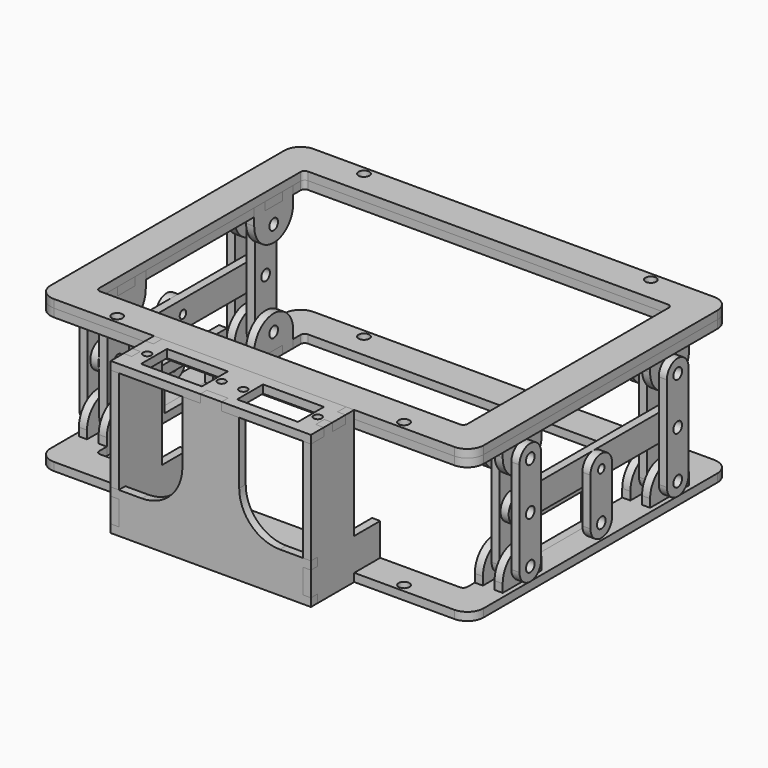
from build123d import *

# Parameters (mm, degrees)
F0_W           = 160
F0_H           = 120
F0_W_2         = 136
F0_H_2         = 96
F1_DEPTH       = 3
F2_R           = 6
F3_R           = 1.5
F4_R           = 2
F5_DEPTH       = 3.001
F6_W           = 2.9
F6_H           = 4.9
F7_DEPTH       = 3.001
F8_R           = 2
F9_DEPTH       = 3
F10_R          = 2
F11_DEPTH      = 3
F18_R          = 2
F19_DEPTH      = 3
F24_R          = 2
F25_DEPTH      = 7
F26_DEPTH      = 4
F30_R          = 1.5
F31_DEPTH      = 158.601
F32_W          = 35.5
F32_H          = 19
F32_R          = 1.5
F32_W_2        = 22.5
F32_H_2        = 12
F33_DEPTH      = 3
F34_W          = 35.3
F34_H          = 3
F35_DEPTH      = 2.9
F35_DEPTH_BACK = 138.9
F36_R          = 2
F36_R_2        = 1.5
F37_DEPTH      = 3
F38_R          = 1.5
F38_W          = 22.5
F38_H          = 12
F39_DEPTH      = 3
F41_DEPTH      = 3
F42_R          = 15
F44_DEPTH      = 3
F45_W          = 3
F45_H          = 4
F46_DEPTH      = 3
F48_R          = 3


with BuildPart() as f1:
    # F0 (on Top) → F1 (new body)
    with BuildSketch(Plane.XY):
        with Locations((-83.0341556995, -58.1203717301)):
            Rectangle(F0_W, F0_H)
        with Locations((-83.0341556995, -58.1203717301)):
            Rectangle(F0_W_2, F0_H_2, mode=Mode.SUBTRACT)
    extrude(amount=F1_DEPTH)

    # F2
    f2_edges = [f1.edges().sort_by_distance(p)[0] for p in [
        (-163.034156, -118.120372, 1.5),
        (-3.034156, -118.120372, 1.5),
        (-163.034156, 1.879628, 1.5),
        (-3.034156, 1.879628, 1.5),
    ]]
    fillet(f2_edges, radius=F2_R)

    # F3
    f3_edges = [f1.edges().sort_by_distance(p)[0] for p in [
        (-151.034156, -10.120372, 1.5),
        (-15.034156, -10.120372, 1.5),
        (-15.034156, -106.120372, 1.5),
        (-151.034156, -106.120372, 1.5),
    ]]
    fillet(f3_edges, radius=F3_R)

    # F4 (on face) → F5 (cut, through all)
    with BuildSketch(Plane.XY.offset(3)):
        with Locations((-136.0341556995, -1.1203717301)):
            Circle(F4_R)
        with Locations((-30.0341556995, -1.1203717301)):
            Circle(F4_R)
        with Locations((-30.0341556995, -115.1203717301)):
            Circle(F4_R)
        with Locations((-136.0341556995, -115.1203717301)):
            Circle(F4_R)
    extrude(amount=-F5_DEPTH, mode=Mode.SUBTRACT)

    # F6 (on face) → F7 (cut, through all)
    with BuildSketch(Plane.XY.offset(3)):
        with Locations((-152.4841556995, -98.6703717301)):
            Rectangle(F6_W, F6_H)
        with Locations((-152.4841556995, -85.6703717301)):
            Rectangle(F6_W, F6_H)
        with Locations((-159.8841556995, -98.6703717301)):
            Rectangle(F6_W, F6_H)
        with Locations((-159.8841556995, -85.6703717301)):
            Rectangle(F6_W, F6_H)
        with Locations((-6.1841556995, -98.6703717301)):
            Rectangle(F6_W, F6_H)
        with Locations((-6.1841556995, -85.6703717301)):
            Rectangle(F6_W, F6_H)
        with Locations((-13.5841556995, -85.6703717301)):
            Rectangle(F6_W, F6_H)
        with Locations((-13.5841556995, -98.6703717301)):
            Rectangle(F6_W, F6_H)
        with Locations((-6.1841556995, -17.5703717301)):
            Rectangle(F6_W, F6_H)
        with Locations((-152.4841556995, -17.5703717301)):
            Rectangle(F6_W, F6_H)
        with Locations((-13.5841556995, -17.5703717301)):
            Rectangle(F6_W, F6_H)
        with Locations((-159.8841556995, -30.5703717301)):
            Rectangle(F6_W, F6_H)
        with Locations((-159.8841556995, -17.5703717301)):
            Rectangle(F6_W, F6_H)
        with Locations((-13.5841556995, -30.5703717301)):
            Rectangle(F6_W, F6_H)
        with Locations((-6.1841556995, -30.5703717301)):
            Rectangle(F6_W, F6_H)
        with Locations((-152.4841556995, -30.5703717301)):
            Rectangle(F6_W, F6_H)
    extrude(amount=-F7_DEPTH, mode=Mode.SUBTRACT)


with BuildPart() as f9:
    # F8 (on face) → F9 (new body)
    with BuildSketch(Plane.XY.offset(3)):
        with BuildLine():
            ThreePointArc((-3.0341556995, -4.1203717301), (-4.7915150124, 0.122268957), (-9.0341556995, 1.8796282699))
            Line((-9.0341556995, 1.8796282699), (-157.0341556995, 1.8796282699))
            ThreePointArc((-157.0341556995, 1.8796282699), (-161.2767963867, 0.122268957), (-163.0341556995, -4.1203717301))
            Line((-163.0341556995, -4.1203717301), (-163.0341556995, -112.1203717301))
            ThreePointArc((-163.0341556995, -112.1203717301), (-161.2767963867, -116.3630124172), (-157.0341556995, -118.1203717301))
            Line((-157.0341556995, -118.1203717301), (-9.0341556995, -118.1203717301))
            ThreePointArc((-9.0341556995, -118.1203717301), (-4.7915150124, -116.3630124172), (-3.0341556995, -112.1203717301))
            Line((-3.0341556995, -112.1203717301), (-3.0341556995, -4.1203717301))
        make_face()
        with Locations((-136.0341556995, -115.1203717301)):
            Circle(F8_R, mode=Mode.SUBTRACT)
        with Locations((-30.0341556995, -115.1203717301)):
            Circle(F8_R, mode=Mode.SUBTRACT)
        with Locations((-136.0341556995, -1.1203717301)):
            Circle(F8_R, mode=Mode.SUBTRACT)
        with BuildLine():
            Line((-16.5341556995, -106.1203717301), (-149.5341556995, -106.1203717301))
            ThreePointArc((-149.5341556995, -106.1203717301), (-150.5948158713, -105.6810319019), (-151.0341556995, -104.6203717301))
            Line((-151.0341556995, -104.6203717301), (-151.0341556995, -11.6203717301))
            ThreePointArc((-151.0341556995, -11.6203717301), (-150.5948158713, -10.5597115583), (-149.5341556995, -10.1203717301))
            Line((-149.5341556995, -10.1203717301), (-16.5341556995, -10.1203717301))
            ThreePointArc((-16.5341556995, -10.1203717301), (-15.4734955278, -10.5597115583), (-15.0341556995, -11.6203717301))
            Line((-15.0341556995, -11.6203717301), (-15.0341556995, -104.6203717301))
            ThreePointArc((-15.0341556995, -104.6203717301), (-15.4734955278, -105.6810319019), (-16.5341556995, -106.1203717301))
        make_face(mode=Mode.SUBTRACT)
        with Locations((-30.0341556995, -1.1203717301)):
            Circle(F8_R, mode=Mode.SUBTRACT)
    extrude(amount=F9_DEPTH)


with BuildPart() as f11:
    # F10 (on face) → F11 (new body)
    with BuildSketch(Plane.YZ.offset(-151.0341556995)):
        with BuildLine():
            Line((-96.2203717301, 3), (-101.1703717301, 3))
            Line((-101.1703717301, 3), (-101.1703717301, -3))
            ThreePointArc((-101.1703717301, -3), (-92.1703717301, -12), (-83.1703717301, -3))
            Line((-83.1703717301, -3), (-83.1703717301, 3))
            Line((-83.1703717301, 3), (-88.1203717301, 3))
            Line((-88.1203717301, 3), (-88.1203717301, 0))
            Line((-88.1203717301, 0), (-88.1703717301, 0))
            Line((-88.1703717301, 0), (-96.1703717301, 0))
            Line((-96.1703717301, 0), (-96.2203717301, 0))
            Line((-96.2203717301, 0), (-96.2203717301, 3))
        make_face()
        with Locations((-92.1703717301, -6)):
            Circle(F10_R, mode=Mode.SUBTRACT)
    extrude(amount=-F11_DEPTH)


with BuildPart() as f13_1:
    # F13: instance of F11
    add(f11.part.mirror(Plane(origin=(-156.1841556995, -71.8953717301, 1.5), x_dir=(0, 1, 0), z_dir=(1, 0, 0))))


with BuildPart() as f16_1:
    # F16: instance of F11
    add(f11.part.mirror(Plane(origin=(-83.0341556995, -58.1203717301, 1.5), x_dir=(0, 1, 0), z_dir=(1, 0, 0))))


with BuildPart() as f16_2:
    # F16: instance of F13_1
    add(f13_1.part.mirror(Plane(origin=(-83.0341556995, -58.1203717301, 1.5), x_dir=(0, 1, 0), z_dir=(1, 0, 0))))


with BuildPart() as f17_1:
    # F17: instance of F11
    add(f11.part.mirror(Plane(origin=(-83.0341556995, -58.1203717301, 1.5), x_dir=(1, 0, 0), z_dir=(0, -1, 0))))


with BuildPart() as f17_2:
    # F17: instance of F13_1
    add(f13_1.part.mirror(Plane(origin=(-83.0341556995, -58.1203717301, 1.5), x_dir=(1, 0, 0), z_dir=(0, -1, 0))))


with BuildPart() as f17_3:
    # F17: instance of F16_1
    add(f16_1.part.mirror(Plane(origin=(-83.0341556995, -58.1203717301, 1.5), x_dir=(1, 0, 0), z_dir=(0, -1, 0))))


with BuildPart() as f17_4:
    # F17: instance of F16_2
    add(f16_2.part.mirror(Plane(origin=(-83.0341556995, -58.1203717301, 1.5), x_dir=(1, 0, 0), z_dir=(0, -1, 0))))


with BuildPart() as f19:
    # F18 (on face) → F19 (new body)
    with BuildSketch(Plane.YZ.offset(-4.7341556995)):
        with BuildLine():
            Line((-87.1703717301, -41), (-87.1703717301, -10.4833147735))
            ThreePointArc((-87.1703717301, -10.4833147735), (-92.1703717301, -12), (-97.1703717301, -10.4833147735))
            Line((-97.1703717301, -10.4833147735), (-97.1703717301, -41))
            ThreePointArc((-97.1703717301, -41), (-92.1703717301, -46), (-87.1703717301, -41))
        make_face()
        with Locations((-92.1703717301, -41)):
            Circle(F18_R, mode=Mode.SUBTRACT)
        with Locations((-92.1703717301, -23.5)):
            Circle(F18_R, mode=Mode.SUBTRACT)
        with BuildLine():
            Line((-87.1703717301, -10.4833147735), (-87.1703717301, -6))
            ThreePointArc((-87.1703717301, -6), (-92.1703717301, -1), (-97.1703717301, -6))
            Line((-97.1703717301, -6), (-97.1703717301, -10.4833147735))
            ThreePointArc((-97.1703717301, -10.4833147735), (-92.1703717301, -12), (-87.1703717301, -10.4833147735))
        make_face()
        with Locations((-92.1703717301, -6)):
            Circle(F18_R, mode=Mode.SUBTRACT)
    extrude(amount=F19_DEPTH)


with BuildPart() as f21_1:
    # F21: instance of F19
    add(f19.part.mirror(Plane(origin=(-6.8841556995, -92.1703717301, -13.8389325215), x_dir=(0, 1, 0), z_dir=(1, 0, 0))))


with BuildPart() as f22_1:
    # F22: instance of F19
    add(f19.part.mirror(Plane(origin=(-83.0341556995, -58.1203717301, 1.5), x_dir=(0, 1, 0), z_dir=(1, 0, 0))))


with BuildPart() as f22_2:
    # F22: instance of F21_1
    add(f21_1.part.mirror(Plane(origin=(-83.0341556995, -58.1203717301, 1.5), x_dir=(0, 1, 0), z_dir=(1, 0, 0))))


with BuildPart() as f23_1:
    # F23: instance of F22_2
    add(f22_2.part.mirror(Plane(origin=(-83.0341556995, -58.1203717301, 1.5), x_dir=(1, 0, 0), z_dir=(0, -1, 0))))


with BuildPart() as f23_2:
    # F23: instance of F19
    add(f19.part.mirror(Plane(origin=(-83.0341556995, -58.1203717301, 1.5), x_dir=(1, 0, 0), z_dir=(0, -1, 0))))


with BuildPart() as f23_3:
    # F23: instance of F22_1
    add(f22_1.part.mirror(Plane(origin=(-83.0341556995, -58.1203717301, 1.5), x_dir=(1, 0, 0), z_dir=(0, -1, 0))))


with BuildPart() as f23_4:
    # F23: instance of F21_1
    add(f21_1.part.mirror(Plane(origin=(-83.0341556995, -58.1203717301, 1.5), x_dir=(1, 0, 0), z_dir=(0, -1, 0))))


with BuildPart() as f25:
    # F24 (on face) → F25 (new body)
    with BuildSketch(Plane.YZ.offset(-1.7341556995)):
        with BuildLine():
            ThreePointArc((-24.0703717301, -28.5), (-19.0703717301, -23.5), (-24.0703717301, -18.5))
            Line((-24.0703717301, -18.5), (-92.1703717301, -18.5))
            ThreePointArc((-92.1703717301, -18.5), (-97.1703717301, -23.5), (-92.1703717301, -28.5))
            Line((-92.1703717301, -28.5), (-24.0703717301, -28.5))
        make_face()
        with Locations((-92.1703717301, -23.5)):
            Circle(F24_R, mode=Mode.SUBTRACT)
        with Locations((-24.0703717301, -23.5)):
            Circle(F24_R, mode=Mode.SUBTRACT)
    extrude(amount=-F25_DEPTH)

    # F24 (on face) → F26 (cut)
    with BuildSketch(Plane.YZ.offset(-1.7341556995)):
        with BuildLine():
            ThreePointArc((-24.0703717301, -28.5), (-19.0703717301, -23.5), (-24.0703717301, -18.5))
            Line((-24.0703717301, -18.5), (-92.1703717301, -18.5))
            ThreePointArc((-92.1703717301, -18.5), (-97.1703717301, -23.5), (-92.1703717301, -28.5))
            Line((-92.1703717301, -28.5), (-24.0703717301, -28.5))
        make_face()
        with Locations((-92.1703717301, -23.5)):
            Circle(F24_R, mode=Mode.SUBTRACT)
        with Locations((-24.0703717301, -23.5)):
            Circle(F24_R, mode=Mode.SUBTRACT)
    extrude(amount=-F26_DEPTH, mode=Mode.SUBTRACT)


with BuildPart() as f27_1:
    # F27: instance of F25
    add(f25.part.mirror(Plane(origin=(-83.0341556995, -58.1203717301, 1.5), x_dir=(0, 1, 0), z_dir=(1, 0, 0))))


with BuildPart() as f29_1:
    # F29: instance of F17_2
    add(f17_2.part.mirror(Plane(origin=(-158.8341556995, -58.1203717301, -23.5), x_dir=(1, 0, 0), z_dir=(0, 0, 1))))


with BuildPart() as f29_2:
    # F29: instance of F13_1
    add(f13_1.part.mirror(Plane(origin=(-158.8341556995, -58.1203717301, -23.5), x_dir=(1, 0, 0), z_dir=(0, 0, 1))))


with BuildPart() as f29_3:
    # F29: instance of F16_2
    add(f16_2.part.mirror(Plane(origin=(-158.8341556995, -58.1203717301, -23.5), x_dir=(1, 0, 0), z_dir=(0, 0, 1))))


with BuildPart() as f29_4:
    # F29: instance of F17_4
    add(f17_4.part.mirror(Plane(origin=(-158.8341556995, -58.1203717301, -23.5), x_dir=(1, 0, 0), z_dir=(0, 0, 1))))


with BuildPart() as f29_5:
    # F29: instance of F1
    add(f1.part.mirror(Plane(origin=(-158.8341556995, -58.1203717301, -23.5), x_dir=(1, 0, 0), z_dir=(0, 0, 1))))

    # F34 (on face) → F35 (cut, two sides)
    with BuildSketch(Plane(origin=(-15.0341556995, 0, 0), x_dir=(0, -1, 0), z_dir=(-1, 0, 0))) as f35_sk:
        with Locations((63.3703717301, -48.5)):
            Rectangle(F34_W, F34_H)
    extrude(amount=-F35_DEPTH, mode=Mode.SUBTRACT)
    extrude(f35_sk.sketch, amount=F35_DEPTH_BACK, mode=Mode.SUBTRACT)

    # F45 (on face) → F46 (cut)
    with BuildSketch(Plane(origin=(0, 0, -50), x_dir=(1, 0, 0), z_dir=(0, 0, -1))):
        with Locations((-118.5341556995, 108.1203717301)):
            Rectangle(F45_W, F45_H)
        with Locations((-47.5341556995, 108.1203717301)):
            Rectangle(F45_W, F45_H)
    extrude(amount=-F46_DEPTH, mode=Mode.SUBTRACT)


with BuildPart() as f29_6:
    # F29: instance of F11
    add(f11.part.mirror(Plane(origin=(-158.8341556995, -58.1203717301, -23.5), x_dir=(1, 0, 0), z_dir=(0, 0, 1))))


with BuildPart() as f29_7:
    # F29: instance of F17_1
    add(f17_1.part.mirror(Plane(origin=(-158.8341556995, -58.1203717301, -23.5), x_dir=(1, 0, 0), z_dir=(0, 0, 1))))


with BuildPart() as f29_8:
    # F29: instance of F17_3
    add(f17_3.part.mirror(Plane(origin=(-158.8341556995, -58.1203717301, -23.5), x_dir=(1, 0, 0), z_dir=(0, 0, 1))))


with BuildPart() as f29_9:
    # F29: instance of F16_1
    add(f16_1.part.mirror(Plane(origin=(-158.8341556995, -58.1203717301, -23.5), x_dir=(1, 0, 0), z_dir=(0, 0, 1))))


with BuildPart() as f31_tool:
    # F30 (on face) → F31 (new body, through all)
    with BuildSketch(Plane.YZ.offset(-5.7341556995)):
        with Locations((-58.1203717301, -23.5)):
            Circle(F30_R)
    extrude(amount=-F31_DEPTH)


with BuildPart() as f25_1:
    add(f25.part)

    # F31: cut by f31_tool
    add(f31_tool.part, mode=Mode.SUBTRACT)


with BuildPart() as f27_1_1:
    add(f27_1.part)

    # F31: cut by f31_tool
    add(f31_tool.part, mode=Mode.SUBTRACT)


with BuildPart() as f33:
    # F32 (on face) → F33 (new body)
    with BuildSketch(Plane(origin=(-15.0341556995, 0, 0), x_dir=(0, -1, 0), z_dir=(-1, 0, 0))):
        with Locations((63.3703717301, -40.5)):
            Rectangle(F32_W, F32_H)
        with Locations((49.6203717301, -41)):
            Circle(F32_R, mode=Mode.SUBTRACT)
        with Locations((63.3703717301, -41)):
            Rectangle(F32_W_2, F32_H_2, mode=Mode.SUBTRACT)
        with Locations((77.1203717301, -41)):
            Circle(F32_R, mode=Mode.SUBTRACT)
    extrude(amount=-F33_DEPTH)


with BuildPart() as f37:
    # F36 (on face) → F37 (new body)
    with BuildSketch(Plane.YZ.offset(-5.7341556995)):
        with BuildLine():
            ThreePointArc((-53.1203717301, -23.5), (-58.1203717301, -18.5), (-63.1203717301, -23.5))
            Line((-63.1203717301, -23.5), (-63.1203717301, -41))
            ThreePointArc((-63.1203717301, -41), (-58.1203717301, -46), (-53.1203717301, -41))
            Line((-53.1203717301, -41), (-53.1203717301, -23.5))
        make_face()
        with Locations((-58.1203717301, -41)):
            Circle(F36_R, mode=Mode.SUBTRACT)
        with Locations((-58.1203717301, -23.5)):
            Circle(F36_R_2, mode=Mode.SUBTRACT)
    extrude(amount=F37_DEPTH)


with BuildPart() as f39:
    # F38 (on face) → F39 (new body)
    with BuildSketch(Plane.XY.offset(6)):
        Polygon((-48.9341556995, -118.1203717301), (-117.1341556995, -118.1203717301), (-117.1341556995, -122.0203717301), (-120.0341556995, -122.0203717301), (-120.0341556995, -128.2203717301), (-117.1341556995, -128.2203717301), (-117.1341556995, -132.1203717301), (-120.0341556995, -132.1203717301), (-120.0341556995, -138.1203717301), (-86.9341556995, -138.1203717301), (-86.9341556995, -135.2203717301), (-79.1341556995, -135.2203717301), (-79.1341556995, -138.1203717301), (-46.0341556995, -138.1203717301), (-46.0341556995, -132.1203717301), (-48.9341556995, -132.1203717301), (-48.9341556995, -128.2203717301), (-46.0341556995, -128.2203717301), (-46.0341556995, -122.0203717301), (-48.9341556995, -122.0203717301), align=None)
        with Locations((-114.5341556995, -128.1203717301)):
            Circle(F38_R, mode=Mode.SUBTRACT)
        with Locations((-100.7841556995, -128.1203717301)):
            Rectangle(F38_W, F38_H, mode=Mode.SUBTRACT)
        with Locations((-87.0341556995, -128.1203717301)):
            Circle(F38_R, mode=Mode.SUBTRACT)
        with Locations((-79.0341556995, -128.1203717301)):
            Circle(F38_R, mode=Mode.SUBTRACT)
        with Locations((-65.2841556995, -128.1203717301)):
            Rectangle(F38_W, F38_H, mode=Mode.SUBTRACT)
        with Locations((-51.5341556995, -128.1203717301)):
            Circle(F38_R, mode=Mode.SUBTRACT)
    extrude(amount=-F39_DEPTH)


with BuildPart() as f41:
    # F40 (on face) → F41 (new body)
    with BuildSketch(Plane.XZ.offset(138.1203717301)):
        Polygon((-120.0341556995, -46.9), (-120.0341556995, -50), (-46.0341556995, -50), (-46.0341556995, -46.9), (-48.9341556995, -46.9), (-48.9341556995, -38.1), (-46.0341556995, -38.1), (-46.0341556995, -35), (-72.5341556995, -35), (-72.5341556995, 3), (-79.0341556995, 3), (-79.0341556995, 6), (-86.9341556995, 6), (-86.9341556995, 3), (-87.0341556995, 3), (-93.5341556995, 3), (-93.5341556995, -35), (-120.0341556995, -35), (-120.0341556995, -38.1), (-117.1341556995, -38.1), (-117.1341556995, -46.9), align=None)
    extrude(amount=-F41_DEPTH)

    # F42
    f42_edges = [f41.edges().sort_by_distance(p)[0] for p in [
        (-93.534156, -136.620372, -35),
        (-72.534156, -136.620372, -35),
    ]]
    fillet(f42_edges, radius=F42_R)


with BuildPart() as f44:
    # F43 (on face) → F44 (new body)
    with BuildSketch(Plane(origin=(-120.0341556995, 0, 0), x_dir=(0, -1, 0), z_dir=(-1, 0, 0))):
        Polygon((118.1203717301, -50), (135.1203717301, -50), (135.1203717301, -47), (138.1203717301, -47), (138.1203717301, -38), (135.1203717301, -38), (135.1203717301, -35), (138.1203717301, -35), (138.1203717301, 3), (132.1703717301, 3), (132.1703717301, 6), (128.1703717301, 6), (128.1703717301, 3), (122.1203717301, 3), (122.1203717301, 6), (118.1203717301, 6), (118.1203717301, 3), (118.1203717301, -35), (106.1203717301, -35), (106.1203717301, -50), (110.1203717301, -50), (110.1203717301, -47), (118.1203717301, -47), align=None)
    extrude(amount=-F44_DEPTH)


with BuildPart() as f47_1:
    # F47: instance of F37
    add(f37.part.mirror(Plane(origin=(-83.0341556995, -58.1203717301, 1.5), x_dir=(0, 1, 0), z_dir=(1, 0, 0))))


with BuildPart() as f47_2:
    # F47: instance of F33
    add(f33.part.mirror(Plane(origin=(-83.0341556995, -58.1203717301, 1.5), x_dir=(0, 1, 0), z_dir=(1, 0, 0))))


with BuildPart() as f47_3:
    # F47: instance of F44
    add(f44.part.mirror(Plane(origin=(-83.0341556995, -58.1203717301, 1.5), x_dir=(0, 1, 0), z_dir=(1, 0, 0))))


with BuildPart() as f33_1:
    add(f33.part)

    # F48
    f48_edges = [f33_1.edges().sort_by_distance(p)[0] for p in [
        (-13.534156, -45.620372, -31),
        (-13.534156, -81.120372, -31),
    ]]
    fillet(f48_edges, radius=F48_R)


solid = Compound([f1.part, f9.part, f11.part, f13_1.part, f16_1.part, f16_2.part, f17_1.part, f17_2.part, f17_3.part, f17_4.part, f19.part, f21_1.part, f22_1.part, f22_2.part, f23_1.part, f23_2.part, f23_3.part, f23_4.part, f29_1.part, f29_2.part, f29_3.part, f29_4.part, f29_5.part, f29_6.part, f29_7.part, f29_8.part, f29_9.part, f25_1.part, f27_1_1.part, f37.part, f39.part, f41.part, f44.part, f47_1.part, f47_2.part, f47_3.part, f33_1.part])
